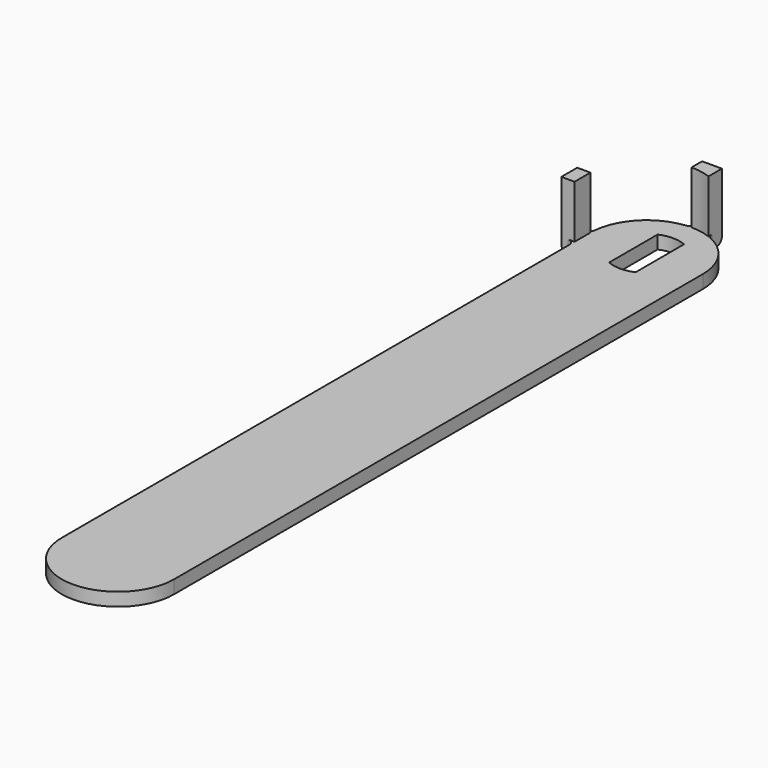
from build123d import *

# Parameters (mm, degrees)
F1_DEPTH = 2
F2_W     = 2
F2_H     = 3
F3_DEPTH = 10
F4_R     = 0.99999


# Not quite as in the source:
# - a fillet or chamfer is up to 0.001 mm smaller than in the source, because OpenCascade refuses the exact size


with BuildPart() as f1:
    # F0 (on Top) → F1 (new body)
    with BuildSketch(Plane.XY):
        with BuildLine():
            Line((8.5, -100), (8.5, 0))
            ThreePointArc((8.5, 0), (0, 8.5), (-8.5, 0))
            Line((-8.5, 0), (-8.5, -100))
            ThreePointArc((-8.5, -100), (0, -108.5), (8.5, -100))
        make_face()
        with BuildLine():
            ThreePointArc((-2, 4.582575695), (0, 5), (2, 4.582575695))
            Line((2, 4.582575695), (2, -4.582575695))
            ThreePointArc((2, -4.582575695), (0, -5), (-2, -4.582575695))
            Line((-2, -4.582575695), (-2, 4.582575695))
        make_face(mode=Mode.SUBTRACT)
    extrude(amount=F1_DEPTH)

    # F2 (on Top) → F3 (join)
    with BuildSketch(Plane.XY):
        with Locations((-9.5, -1.5)):
            Rectangle(F2_W, F2_H)
        with BuildLine():
            Line((0, 10.5), (0, 8.5))
            ThreePointArc((0, 8.5), (1.5247314005, 8.3621285661), (3, 7.9529868603))
            Line((3, 7.9529868603), (3, 10.5))
            Line((3, 10.5), (0, 10.5))
        make_face()
    extrude(amount=F3_DEPTH)

    # F4 (radius 1 in the source; OpenCascade refuses exactly that, so slightly less here)
    f4_edges = [f1.edges().sort_by_distance(p)[0] for p in [
        (-8.5, 0, 1),
        (0, 8.5, 1),
        (-8.5, -3, 1),
        (-10.5, -1.5, 0),
        (1.5, 10.5, 0),
        (3, 7.952987, 1),
    ]]
    fillet(f4_edges, radius=F4_R)


solid = f1.part
